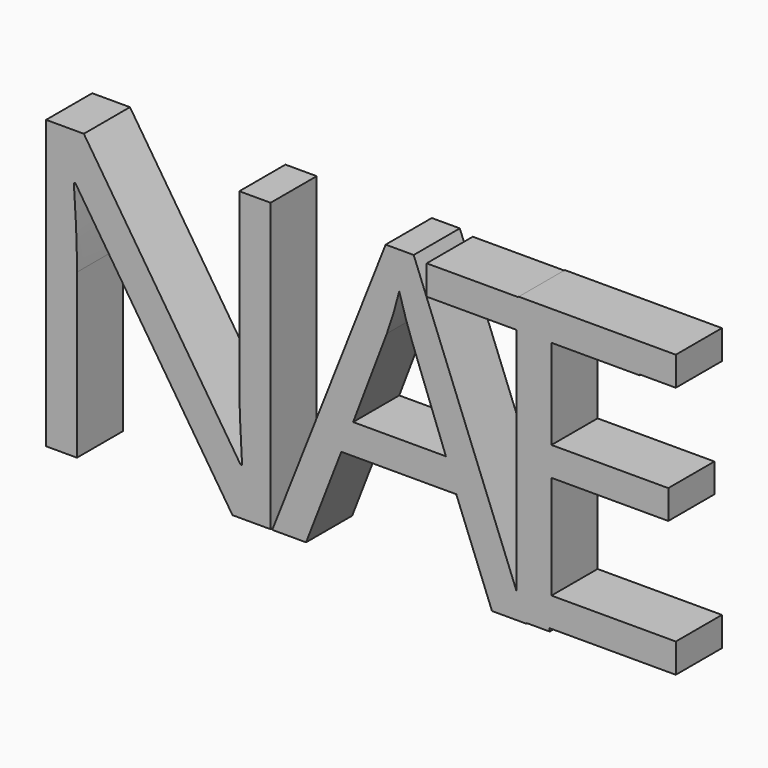
from build123d import *

# Parameters (mm, degrees)
F0_TEXT_SIZE = 177.0021600856
F3_DEPTH     = 25.4
F1_TEXT_SIZE = 175.3957528207
F4_DEPTH     = 25.4
F2_TEXT_SIZE = 173.9093412956
F5_DEPTH     = 25.4
F6_TEXT_SIZE = 177.3832779792
F7_DEPTH     = 25.4


# Not quite as in the source:
# - Text() gives the source's letters only with a copy of the font that has no kerning and outlines rounded to 1/6400 em; it was checked with that copy


with BuildPart() as f3:
    # F0 (on Front) → F3 (new body)
    with BuildSketch(Plane.XZ):
        with Locations((3.9664511569, -64.606718719)):
            Text('A', F0_TEXT_SIZE, font='Open Sans', text_align=(TextAlign.LEFT, TextAlign.BOTTOM))
    extrude(amount=F3_DEPTH)

    # F1 (on Front) → F4 (join)
    with BuildSketch(Plane.XZ):
        with Locations((70.4521909356, -64.3124803901)):
            Text('T', F1_TEXT_SIZE, font='Open Sans', text_align=(TextAlign.LEFT, TextAlign.BOTTOM))
    extrude(amount=F4_DEPTH)

    # F2 (on Front) → F5 (join)
    with BuildSketch(Plane.XZ):
        with Locations((95.482237637, -63.0008848384)):
            Text('E', F2_TEXT_SIZE, font='Open Sans', text_align=(TextAlign.LEFT, TextAlign.BOTTOM))
    extrude(amount=F5_DEPTH)


with BuildPart() as f7:
    # F6 (on Front) → F7 (new body)
    with BuildSketch(Plane.XZ):
        with Locations((-113.1081450731, -64.606718719)):
            Text('N', F6_TEXT_SIZE, font='Open Sans', text_align=(TextAlign.LEFT, TextAlign.BOTTOM))
    extrude(amount=F7_DEPTH)


solid = Compound([f3.part, f7.part])
